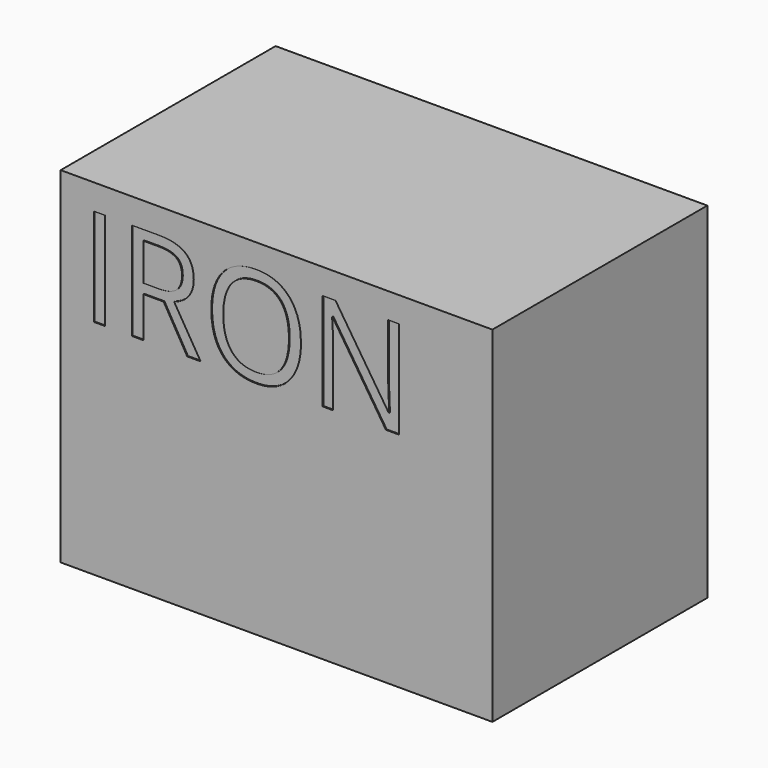
from build123d import *

# Parameters (mm, degrees)
F0_W         = 450
F0_H         = 280
F1_DEPTH     = 360
F2_TEXT_SIZE = 142.3323733939
F3_DEPTH     = 1


# Not quite as in the source:
# - Text() gives the source's letters only with a copy of the font that has no kerning and outlines rounded to 1/6400 em; it was checked with that copy


with BuildPart() as f1:
    # F0 (on Top) → F1 (new body)
    with BuildSketch(Plane.XY):
        Rectangle(F0_W, F0_H)
    extrude(amount=F1_DEPTH)

    # F2 (on face) → F3 (cut)
    with BuildSketch(Plane.XZ.offset(140)):
        with Locations((-204.3659836054, 231.9343388081)):
            Text('IRON', F2_TEXT_SIZE, font='Open Sans', text_align=(TextAlign.LEFT, TextAlign.BOTTOM))
    extrude(amount=-F3_DEPTH, mode=Mode.SUBTRACT)


solid = f1.part
